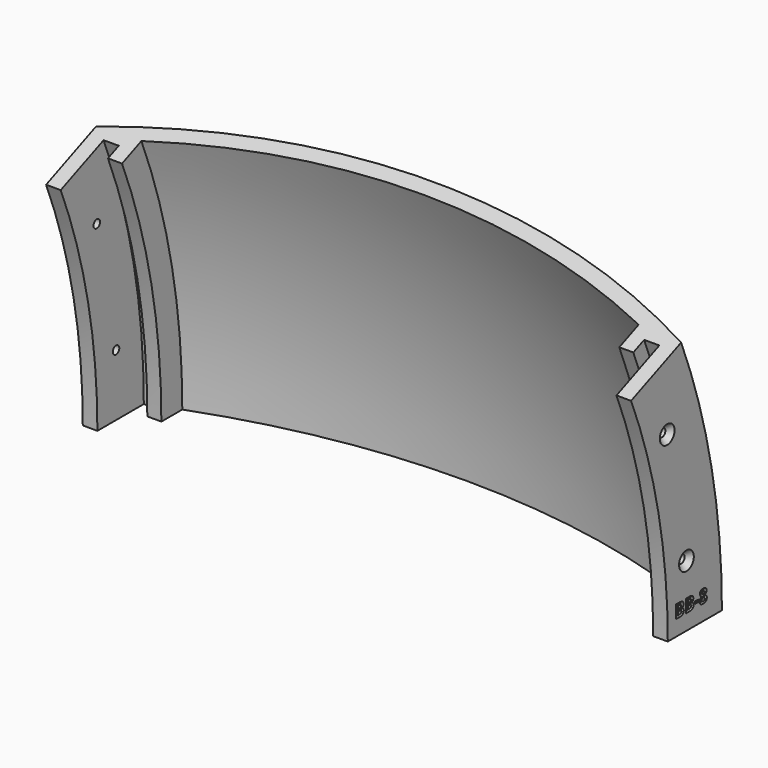
from build123d import *

# Parameters (mm, degrees)
F1_ANGLE     = 22.5
F2_R         = 1.4
F3_DEPTH     = 139.36235
F4_TEXT_SIZE = 6.2362746879
F5_DEPTH     = 1
F6_SIZE      = 1.75


# Not quite as in the source:
# - a feature names something its author has since deleted; it is built from what else it names
# - Text() gives the source's letters only with a copy of the font that has no kerning and outlines rounded to 1/6400 em; it was checked with that copy


with BuildPart() as f1:
    # F0 (on Top) → F1 (revolve)
    with BuildSketch(Plane.XY):
        with BuildLine():
            Line((-95, 206), (-95, 225.8317958127))
            ThreePointArc((-95, 225.8317958127), (-90.0216753203, 227.8620152033), (-85, 229.7825058615))
            ThreePointArc((-85, 229.7825058615), (0, 245), (85, 229.7825058615))
            ThreePointArc((85, 229.7825058615), (90.0216753203, 227.8620152033), (95, 225.8317958127))
            Line((95, 225.8317958127), (95, 206))
            Line((95, 206), (100, 206))
            Line((100, 206), (100, 229.1287847478))
            ThreePointArc((100, 229.1287847478), (0, 250), (-100, 229.1287847478))
            Line((-100, 229.1287847478), (-100, 206))
            Line((-100, 206), (-95, 206))
        make_face()
        with BuildLine():
            ThreePointArc((-85, 229.7825058615), (-90.0216753203, 227.8620152033), (-95, 225.8317958127))
            Line((-95, 225.8317958127), (-89.8, 225.8317958127))
            Line((-89.8, 225.8317958127), (-89.8, 220.8317958127))
            Line((-89.8, 220.8317958127), (-85, 220.8317958127))
            Line((-85, 220.8317958127), (-85, 229.7825058615))
        make_face()
        with BuildLine():
            ThreePointArc((95, 225.8317958127), (90.0216753203, 227.8620152033), (85, 229.7825058615))
            Line((85, 229.7825058615), (85, 220.8317958127))
            Line((85, 220.8317958127), (89.8, 220.8317958127))
            Line((89.8, 220.8317958127), (89.8, 225.8317958127))
            Line((89.8, 225.8317958127), (95, 225.8317958127))
        make_face()
    revolve(axis=Axis((0, 0, 0), (1, 0, 0)), revolution_arc=F1_ANGLE)

    # F2 (on Right) → F3 (cut, symmetric)
    with BuildSketch(Plane.YZ):
        with Locations((205.7421721824, 62.4112056097)):
            Circle(F2_R)
        with Locations((213.9647162345, 21.0736851709)):
            Circle(F2_R)
    extrude(amount=F3_DEPTH, both=True, mode=Mode.SUBTRACT)

    # F4 (on face) → F5 (cut)
    with BuildSketch(Plane.YZ.offset(100)):
        with Locations((208.9602351189, 5.3157305811)):
            Text('BB-8', F4_TEXT_SIZE, font='Open Sans', font_style=FontStyle.BOLD, text_align=(TextAlign.LEFT, TextAlign.BOTTOM))
    extrude(amount=-F5_DEPTH, mode=Mode.SUBTRACT)

    # F6
    f6_edges = [f1.edges().sort_by_distance(p)[0] for p in [
        (100, 212.564716, 21.073685),
        (100, 204.342172, 62.411206),
        (-100, 212.564716, 21.073685),
        (-100, 204.342172, 62.411206),
    ]]
    chamfer(f6_edges, length=F6_SIZE)


solid = f1.part
